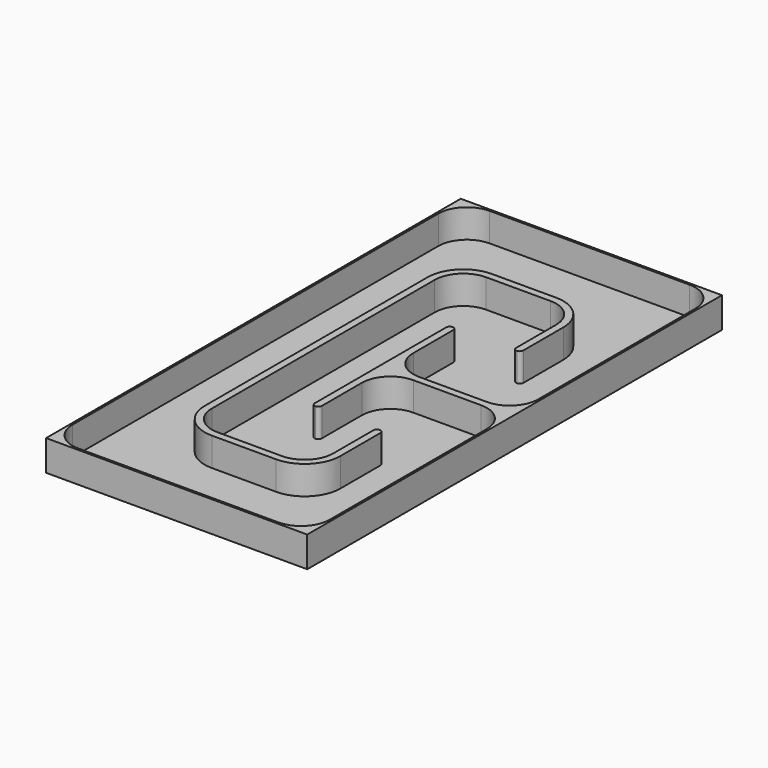
from build123d import *

# Parameters (mm, degrees)
F6_W          = 1828
F6_H          = 3628
F7_DEPTH      = 200
F7_DEPTH_BACK = 14
F8_T          = -14
F11_W         = 50
F11_H         = 200
F16_R         = 200
F16_2_R       = 200
F17_R         = 250
F18_R         = 24.99999
F18_2_R       = 24.99999


# Not quite as in the source:
# - a fillet or chamfer is up to 0.001 mm smaller than in the source, because OpenCascade refuses the exact size


with BuildPart() as f7:
    # F6 (on Top) → F7 (new body, two sides)
    with BuildSketch(Plane.XY) as f7_sk:
        Rectangle(F6_W, F6_H)
    extrude(amount=F7_DEPTH)
    extrude(f7_sk.sketch, amount=-F7_DEPTH_BACK)

    # F8
    f8_openings = [f7.faces().sort_by_distance(p)[0] for p in [
        (0, 0, 200),
    ]]
    offset(amount=F8_T, openings=f8_openings)


with BuildPart() as f12:
    # F12: sweep along a path in F9
    with BuildLine(Plane.XY) as f12_path:
        Line((450, 600), (450, 1200))
        Line((450, 1200), (-450, 1200))
        Line((-450, 1200), (-450, 0))
        Line((-450, 0), (-450, -1200))
        Line((-450, -1200), (450, -1200))
        Line((450, -1200), (450, -600))
    # F11 (on plane+point) → F12 (sweep)
    with BuildSketch(Plane.XZ.offset(-600)):
        with Locations((450, 100)):
            Rectangle(F11_W, F11_H)
    sweep(path=f12_path.line, transition=Transition.RIGHT)

    # F16
    f16_edges = [f12.edges().sort_by_distance(p)[0] for p in [
        (-425, 1175, 100),
        (425, 1175, 100),
        (-425, -1175, 100),
        (425, -1175, 100),
    ]]
    fillet(f16_edges, radius=F16_R)

    # F17
    f17_edges = [f12.edges().sort_by_distance(p)[0] for p in [
        (-475, 1225, 100),
        (475, 1225, 100),
        (-475, -1225, 100),
        (475, -1225, 100),
    ]]
    fillet(f17_edges, radius=F17_R)

    # F18 (radius 25 in the source; OpenCascade refuses exactly that, so slightly less here)
    f18_edges = [f12.edges().sort_by_distance(p)[0] for p in [
        (425, 600, 100),
        (475, 600, 100),
        (425, -600, 100),
        (475, -600, 100),
    ]]
    fillet(f18_edges, radius=F18_R)


with BuildPart() as f13:
    # F13: sweep along a path in F9
    with BuildLine(Plane.XY) as f13_path:
        Line((0, 600), (0, 0))
        Line((0, 0), (900, 0))
    # F11 (on plane+point) → F13 (sweep)
    with BuildSketch(Plane.XZ.offset(-600)):
        with Locations((0, 100)):
            Rectangle(F11_W, F11_H)
    sweep(path=f13_path.line, transition=Transition.RIGHT)


with BuildPart() as f14:
    # F14: sweep along a path in F9
    with BuildLine(Plane.XY) as f14_path:
        Line((0, 600), (0, 0))
        Line((0, 0), (0, -600))
    # F11 (on plane+point) → F14 (sweep)
    with BuildSketch(Plane.XZ.offset(-600)):
        with Locations((0, 100)):
            Rectangle(F11_W, F11_H)
    sweep(path=f14_path.line)


with BuildPart() as f7_1:
    add(f7.part)

    # F15: union F13, F14
    add(f13.part)
    add(f14.part)

    # F16#2
    f16_2_edges = [f7_1.edges().sort_by_distance(p)[0] for p in [
        (25, 25, 100),
        (25, -25, 100),
        (900, -1800, 100),
        (-900, -1800, 100),
        (-900, 1800, 100),
        (900, 1800, 100),
        (900, -25, 100),
        (900, 25, 100),
    ]]
    fillet(f16_2_edges, radius=F16_2_R)

    # F18#2 (radius 25 in the source; OpenCascade refuses exactly that, so slightly less here)
    f18_2_edges = [f7_1.edges().sort_by_distance(p)[0] for p in [
        (-25, 600, 100),
        (25, 600, 100),
        (-25, -600, 100),
        (25, -600, 100),
    ]]
    fillet(f18_2_edges, radius=F18_2_R)


solid = Compound([f12.part, f7_1.part])
